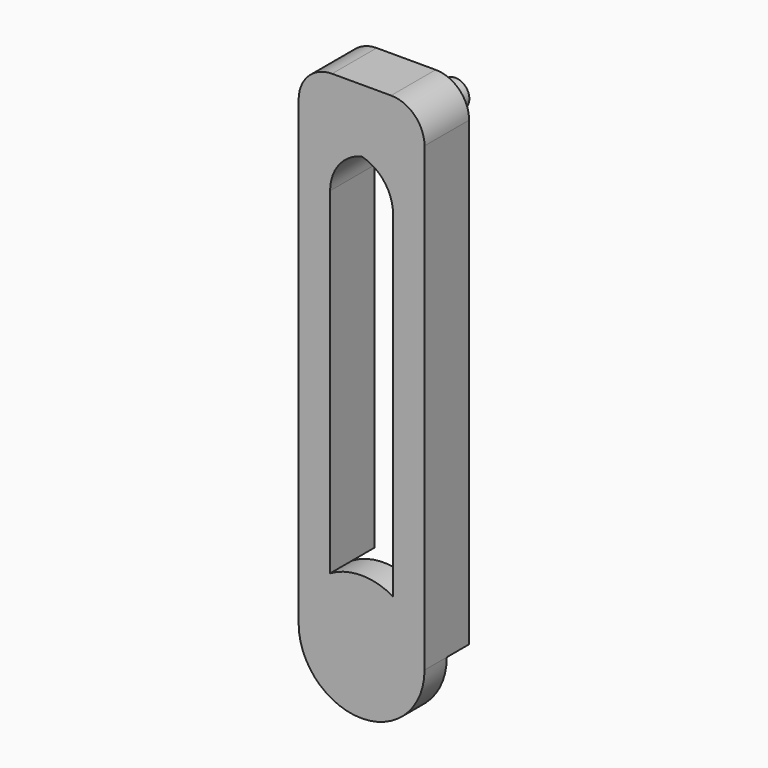
from build123d import *

# Parameters (mm, degrees)
F1_DEPTH    = 1.27
F3_R        = 1.524
F5_T1_DEPTH = 1.27
F2_R        = 1.2397519619
F6_DEPTH    = 2.1971
F4_R        = 0.6356353333
F4_R_2      = 0.6409754112
F7_DEPTH    = 3.429
F9_DEPTH    = 2.54


# Not quite as in the source:
# - a fillet or chamfer that OpenCascade refuses, or shapes differently, is made with other operations: its cross-section is extruded or revolved along the edge and cut away or added


with BuildPart() as f1:
    # F0 (on Front) → F1 (new body)
    with BuildSketch(Plane.XZ):
        with BuildLine():
            ThreePointArc((1.4341250062, 5.3522273875), (2.4839773751, 4.3023750186), (2.8682500124, 2.8682500124))
            Line((2.8682500124, 2.8682500124), (2.8682500124, 25.4276227206))
            Line((2.8682500124, 25.4276227206), (0, 25.4276227206))
            Line((0, 25.4276227206), (-1.4341250062, 25.4276227206))
            Line((-1.4341250062, 25.4276227206), (-2.8682500124, 25.4276227206))
            Line((-2.8682500124, 25.4276227206), (-2.8682500124, 2.8682500124))
            ThreePointArc((-2.8682500124, 2.8682500124), (-2.4839773751, 4.3023750186), (-1.4341250062, 5.3522273875))
            Line((-1.4341250062, 5.3522273875), (-1.4341250062, 22.6080268621))
            Line((-1.4341250062, 22.6080268621), (1.4341250062, 22.6080268621))
            Line((1.4341250062, 22.6080268621), (1.4341250062, 5.3522273875))
        make_face()
        with BuildLine():
            ThreePointArc((-2.8682500124, 2.8682500124), (0, 0), (2.8682500124, 2.8682500124))
            ThreePointArc((2.8682500124, 2.8682500124), (2.4839773751, 4.3023750186), (1.4341250062, 5.3522273875))
            ThreePointArc((1.4341250062, 5.3522273875), (0, 5.7365000248), (-1.4341250062, 5.3522273875))
            ThreePointArc((-1.4341250062, 5.3522273875), (-2.4839773751, 4.3023750186), (-2.8682500124, 2.8682500124))
        make_face()
    extrude(amount=F1_DEPTH)

    # F3
    f3_edges = [f1.edges().sort_by_distance(p)[0] for p in [
        (2.86825, -0.635, 25.427623),
        (-2.86825, -0.635, 25.427623),
    ]]
    fillet(f3_edges, radius=F3_R)

    # F5: fillet of radius 1.905 on 2 edges, made by hand

    # F5_s2 → F5_t1 (join)
    with BuildSketch(Plane.XZ):
        with BuildLine():
            ThreePointArc((-0.4708749938, 22.6080268621), (0.8761634244, 22.0500652803), (1.4341250062, 20.7030268621))
            Line((1.4341250062, 20.7030268621), (1.4341250062, 22.6080268621))
            Line((1.4341250062, 22.6080268621), (-0.4708749938, 22.6080268621))
        make_face()
        with BuildLine():
            ThreePointArc((-1.4341250062, 20.7030268621), (-0.8761634244, 22.0500652803), (0.4708749938, 22.6080268621))
            Line((0.4708749938, 22.6080268621), (-1.4341250062, 22.6080268621))
            Line((-1.4341250062, 22.6080268621), (-1.4341250062, 20.7030268621))
        make_face()
    extrude(amount=F5_T1_DEPTH)

    # F2 (on face) → F6 (join)
    with BuildSketch(Plane(origin=(0, 0, 0), x_dir=(-1, 0, 0), z_dir=(0, 1, 0))):
        with Locations((0, 2.8682500124)):
            Circle(F2_R)
    extrude(amount=F6_DEPTH)

    # F4 (on face) → F7 (join)
    with BuildSketch(Plane.XZ.offset(1.27)):
        with Locations((-1.5970880988, 24.1730304042)):
            Circle(F4_R)
        with Locations((1.5335635452, 24.1730304042)):
            Circle(F4_R)
        with Locations((0, 23.8491314396)):
            Circle(F4_R_2)
    extrude(amount=-F7_DEPTH)

    # F8 (on face) → F9 (join)
    with BuildSketch(Plane.XZ.offset(1.27)):
        with BuildLine():
            ThreePointArc((1.4341250062, 5.3522273875), (2.4839773751, 4.3023750186), (2.8682500124, 2.8682500124))
            Line((2.8682500124, 2.8682500124), (2.8682500124, 23.9036227206))
            ThreePointArc((2.8682500124, 23.9036227206), (1.7143439066, 22.42524303), (0, 23.1855921473))
            ThreePointArc((0, 23.1855921473), (-1.7143439066, 22.42524303), (-2.8682500124, 23.9036227206))
            Line((-2.8682500124, 23.9036227206), (-2.8682500124, 22.548914654))
            Line((-2.8682500124, 22.548914654), (-2.8682500124, 2.8682500124))
            ThreePointArc((-2.8682500124, 2.8682500124), (-2.4839773751, 4.3023750186), (-1.4341250062, 5.3522273875))
            Line((-1.4341250062, 5.3522273875), (-1.4341250062, 20.7030268621))
            ThreePointArc((-1.4341250062, 20.7030268621), (-1.0334590554, 21.8717886293), (0, 22.548914654))
            ThreePointArc((0, 22.548914654), (1.0334590554, 21.8717886293), (1.4341250062, 20.7030268621))
            Line((1.4341250062, 20.7030268621), (1.4341250062, 5.3522273875))
        make_face()
        with BuildLine():
            ThreePointArc((-2.8682500124, 23.9036227206), (-1.7143439066, 22.42524303), (0, 23.1855921473))
            ThreePointArc((0, 23.1855921473), (-0.1797499876, 23.9036227206), (0, 24.6216532939))
            ThreePointArc((0, 24.6216532939), (-0.5605736103, 25.2106909273), (-1.3442500124, 25.4276227206))
            ThreePointArc((-1.3442500124, 25.4276227206), (-2.4218807469, 24.9812534551), (-2.8682500124, 23.9036227206))
        make_face()
        with BuildLine():
            ThreePointArc((0, 23.1855921473), (1.7143439066, 22.42524303), (2.8682500124, 23.9036227206))
            ThreePointArc((2.8682500124, 23.9036227206), (2.4218807469, 24.9812534551), (1.3442500124, 25.4276227206))
            ThreePointArc((1.3442500124, 25.4276227206), (0.5605736103, 25.2106909273), (0, 24.6216532939))
            ThreePointArc((0, 24.6216532939), (0.1341296782, 24.2737166148), (0.1797499876, 23.9036227206))
            ThreePointArc((0.1797499876, 23.9036227206), (0.1341296782, 23.5335288264), (0, 23.1855921473))
        make_face()
        with BuildLine():
            ThreePointArc((0, 24.6216532939), (-0.1797499876, 23.9036227206), (0, 23.1855921473))
            ThreePointArc((0, 23.1855921473), (0.1341296782, 23.5335288264), (0.1797499876, 23.9036227206))
            ThreePointArc((0.1797499876, 23.9036227206), (0.1341296782, 24.2737166148), (0, 24.6216532939))
        make_face()
        with BuildLine():
            ThreePointArc((0, 24.6216532939), (0.5605736103, 25.2106909273), (1.3442500124, 25.4276227206))
            Line((1.3442500124, 25.4276227206), (-1.3442500124, 25.4276227206))
            ThreePointArc((-1.3442500124, 25.4276227206), (-0.5605736103, 25.2106909273), (0, 24.6216532939))
        make_face()
    extrude(amount=-F9_DEPTH)


solid = f1.part
